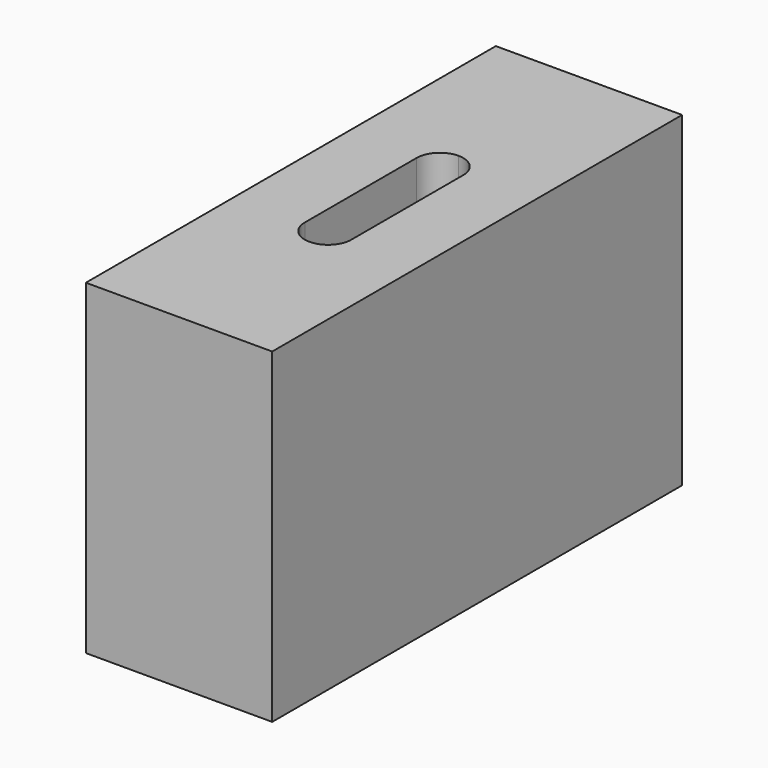
from build123d import *

# Parameters (mm, degrees)
F0_W     = 20
F0_H     = 55
F1_DEPTH = 35
F2_W     = 5
F2_H     = 20
F3_DEPTH = 35.001
F4_R     = 2.49999


# Not quite as in the source:
# - a fillet or chamfer is up to 0.001 mm smaller than in the source, because OpenCascade refuses the exact size


with BuildPart() as f1:
    # F0 (on Top) → F1 (new body)
    with BuildSketch(Plane.XY):
        Rectangle(F0_W, F0_H)
    extrude(amount=F1_DEPTH)

    # F2 (on face) → F3 (cut, through all)
    with BuildSketch(Plane.XY.offset(35)):
        Rectangle(F2_W, F2_H)
    extrude(amount=-F3_DEPTH, mode=Mode.SUBTRACT)

    # F4 (radius 2.5 in the source; OpenCascade refuses exactly that, so slightly less here)
    f4_edges = [f1.edges().sort_by_distance(p)[0] for p in [
        (-2.5, 10, 17.5),
        (2.5, 10, 17.5),
        (2.5, -10, 17.5),
        (-2.5, -10, 17.5),
    ]]
    fillet(f4_edges, radius=F4_R)


solid = f1.part
